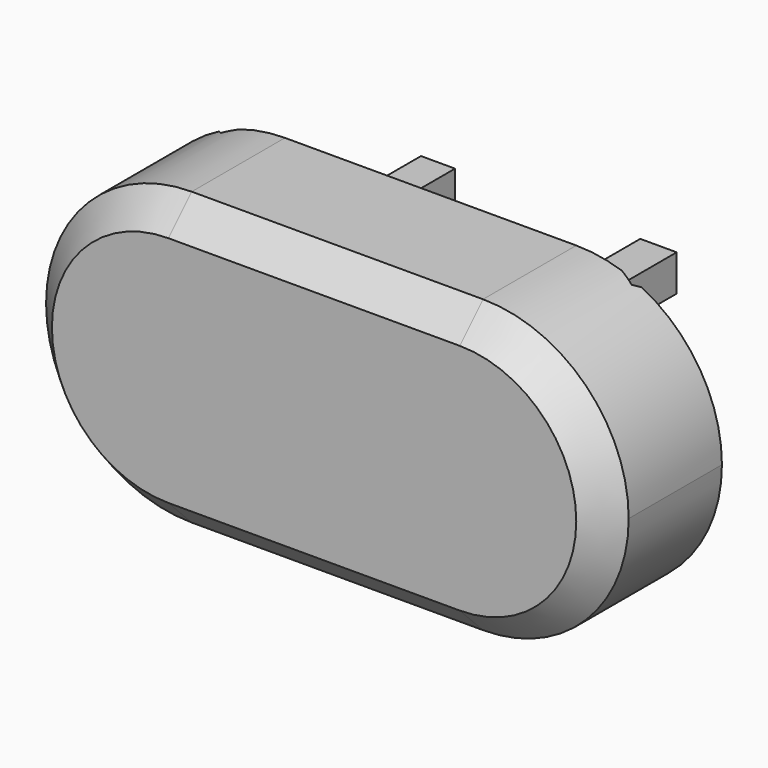
from build123d import *

# Parameters (mm, degrees)
F1_DEPTH     = 25.4
F2_W         = 63.5
F2_H         = 38.1
F3_DEPTH     = 12.7
F4_T1_DEPTH  = 63.5
F4_T3_DEPTH  = 38.1
F4_T5_DEPTH  = 50.8
F4_T8_ANGLE  = 180
F4_T10_ANGLE = 180
F4_T15_DEPTH = 76.5641495789
F4_S16_R     = 25.4
F4_T17_DEPTH = 40
F4_T21_DEPTH = 51.1641495789
F4_S22_R     = 25.4
F4_T23_DEPTH = 27
F4_T30_DEPTH = 76.5641495789
F4_S31_R     = 25.4
F4_T32_DEPTH = 40
F4_T36_DEPTH = 51.1641495789
F4_S37_R     = 25.4
F4_T38_DEPTH = 27
F4_T45_DEPTH = 51.1641495789
F4_S46_R     = 25.4
F4_T47_DEPTH = 27
F4_T51_DEPTH = 76.5641495789
F4_S52_R     = 25.4
F4_T53_DEPTH = 40
F4_T60_DEPTH = 76.5641495789
F4_S61_R     = 25.4
F4_T62_DEPTH = 40
F4_T66_DEPTH = 51.1641495789
F4_S67_R     = 25.4
F4_T68_DEPTH = 27
F5_W         = 6.35
F5_H         = 6.35
F5_W_2       = 5.9358693383
F5_H_2       = 6.4880426841
F5_W_3       = 5.79782274
F5_H_3       = 5.521739329
F5_W_4       = 5.9358680336
F5_H_4       = 6.6260866729
F6_DEPTH     = 25.4


# Not quite as in the source:
# - a fillet or chamfer that OpenCascade refuses, or shapes differently, is made with other operations: its cross-section is extruded or revolved along the edge and cut away or added


with BuildPart() as f1:
    # F0 (on Front) → F1 (new body)
    with BuildSketch(Plane.XZ):
        with BuildLine():
            ThreePointArc((-50.8, 0), (-43.3605122421, -17.9605122421), (-25.4, -25.4))
            Line((-25.4, -25.4), (25.4, -25.4))
            ThreePointArc((25.4, -25.4), (43.3605122421, -17.9605122421), (50.8, 0))
            ThreePointArc((50.8, 0), (43.3605122421, 17.9605122421), (25.4, 25.4))
            Line((25.4, 25.4), (-25.4, 25.4))
            ThreePointArc((-25.4, 25.4), (-43.3605122421, 17.9605122421), (-50.8, 0))
        make_face()
    extrude(amount=F1_DEPTH)

    # F2 (on Front) → F3 (cut)
    with BuildSketch(Plane.XZ):
        Rectangle(F2_W, F2_H)
    extrude(amount=F3_DEPTH, mode=Mode.SUBTRACT)

    # F4: chamfer of 5.08 on 8 edges, made by hand

    # F4_s2 → F4_t1 (cut)
    with BuildSketch(Plane.YZ.offset(-31.75)):
        Polygon((0, 24.13), (-5.08, 19.05), (0, 19.05), align=None)
        Polygon((0, -24.13), (-5.08, -19.05), (0, -19.05), align=None)
    extrude(amount=F4_T1_DEPTH, mode=Mode.SUBTRACT)

    # F4_s4 → F4_t3 (cut)
    with BuildSketch(Plane.XY.offset(-19.05)):
        Polygon((-36.83, 0), (-31.75, -5.08), (-31.75, 0), align=None)
        Polygon((36.83, 0), (31.75, -5.08), (31.75, 0), align=None)
    extrude(amount=F4_T3_DEPTH, mode=Mode.SUBTRACT)

    # F4_s6 → F4_t5 (cut)
    with BuildSketch(Plane.YZ.offset(-25.4)):
        Polygon((-20.32, 25.4), (-25.4, 20.32), (-25.4, 25.4), align=None)
        Polygon((-25.4, -20.32), (-20.32, -25.4), (-25.4, -25.4), align=None)
    extrude(amount=F4_T5_DEPTH, mode=Mode.SUBTRACT)

    # F4_s7 → F4_t8 (revolve, cut)
    with BuildSketch(Plane.YZ.offset(-25.4)):
        Polygon((-20.32, -25.4), (-25.4, -20.32), (-25.4, -25.4), align=None)
    revolve(axis=Axis((-25.4, -25.4, 0), (0, 1, 0)), revolution_arc=F4_T8_ANGLE, mode=Mode.SUBTRACT)

    # F4_s9 → F4_t10 (revolve, cut)
    with BuildSketch(Plane.YZ.offset(25.4)):
        Polygon((-25.4, 20.32), (-20.32, 25.4), (-25.4, 25.4), align=None)
    revolve(axis=Axis((25.4, -25.4, 0), (0, 1, 0)), revolution_arc=F4_T10_ANGLE, mode=Mode.SUBTRACT)


with BuildPart() as f4_tool13:
    # F4_s14 → F4_t15 (new body)
    with BuildSketch(Plane.YZ.offset(44.8141495789)):
        Polygon((0, 24.13), (-5.08, 19.05), (0, 19.05), align=None)
    extrude(amount=-F4_T15_DEPTH)

    # F4_s16 → F4_t17 (intersect, symmetric)
    with BuildSketch(Plane.XZ.offset(2.5)):
        with Locations((25.4, 0)):
            Circle(F4_S16_R)
    extrude(amount=F4_T17_DEPTH, both=True, mode=Mode.INTERSECT)

    split(bisect_by=Plane.YZ.offset(31.75), keep=Keep.TOP)


with BuildPart() as f4_tool19:
    # F4_s20 → F4_t21 (new body)
    with BuildSketch(Plane.XY.offset(-19.05)):
        Polygon((36.83, 0), (31.75, -5.08), (31.75, 0), align=None)
    extrude(amount=F4_T21_DEPTH)

    # F4_s22 → F4_t23 (intersect, symmetric)
    with BuildSketch(Plane.XZ.offset(2.5)):
        with Locations((25.4, 0)):
            Circle(F4_S22_R)
    extrude(amount=F4_T23_DEPTH, both=True, mode=Mode.INTERSECT)

    split(bisect_by=Plane.XY.offset(19.05), keep=Keep.TOP)


with BuildPart() as f4_tool13_1:
    add(f4_tool13.part)

    # F4_t25: intersect F4_tool19
    add(f4_tool19.part, mode=Mode.INTERSECT)


with BuildPart() as f1_1:
    add(f1.part)

    # F4_t11: cut F4_tool13
    add(f4_tool13_1.part, mode=Mode.SUBTRACT)


with BuildPart() as f4_tool28:
    # F4_s29 → F4_t30 (new body)
    with BuildSketch(Plane.YZ.offset(31.75)):
        Polygon((0, 24.13), (-5.08, 19.05), (0, 19.05), align=None)
    extrude(amount=-F4_T30_DEPTH)

    # F4_s31 → F4_t32 (intersect, symmetric)
    with BuildSketch(Plane.XZ.offset(2.5)):
        with Locations((-25.4, 0)):
            Circle(F4_S31_R)
    extrude(amount=F4_T32_DEPTH, both=True, mode=Mode.INTERSECT)

    split(bisect_by=Plane.YZ.offset(-31.75), keep=Keep.BOTTOM)


with BuildPart() as f4_tool34:
    # F4_s35 → F4_t36 (new body)
    with BuildSketch(Plane.XY.offset(32.1141495789)):
        Polygon((-36.83, 0), (-31.75, -5.08), (-31.75, 0), align=None)
    extrude(amount=-F4_T36_DEPTH)

    # F4_s37 → F4_t38 (intersect, symmetric)
    with BuildSketch(Plane.XZ.offset(2.5)):
        with Locations((-25.4, 0)):
            Circle(F4_S37_R)
    extrude(amount=F4_T38_DEPTH, both=True, mode=Mode.INTERSECT)

    split(bisect_by=Plane.XY.offset(19.05), keep=Keep.TOP)


with BuildPart() as f4_tool28_1:
    add(f4_tool28.part)

    # F4_t40: intersect F4_tool34
    add(f4_tool34.part, mode=Mode.INTERSECT)


with BuildPart() as f1_2:
    add(f1_1.part)

    # F4_t26: cut F4_tool28
    add(f4_tool28_1.part, mode=Mode.SUBTRACT)


with BuildPart() as f4_tool43:
    # F4_s44 → F4_t45 (new body)
    with BuildSketch(Plane.XY.offset(19.05)):
        Polygon((-36.83, 0), (-31.75, -5.08), (-31.75, 0), align=None)
    extrude(amount=-F4_T45_DEPTH)

    # F4_s46 → F4_t47 (intersect, symmetric)
    with BuildSketch(Plane.XZ.offset(2.5)):
        with Locations((-25.4, 0)):
            Circle(F4_S46_R)
    extrude(amount=F4_T47_DEPTH, both=True, mode=Mode.INTERSECT)

    split(bisect_by=Plane.XY.offset(-19.05), keep=Keep.BOTTOM)


with BuildPart() as f4_tool49:
    # F4_s50 → F4_t51 (new body)
    with BuildSketch(Plane.YZ.offset(-44.8141495789)):
        Polygon((0, -24.13), (-5.08, -19.05), (0, -19.05), align=None)
    extrude(amount=F4_T51_DEPTH)

    # F4_s52 → F4_t53 (intersect, symmetric)
    with BuildSketch(Plane.XZ.offset(2.5)):
        with Locations((-25.4, 0)):
            Circle(F4_S52_R)
    extrude(amount=F4_T53_DEPTH, both=True, mode=Mode.INTERSECT)

    split(bisect_by=Plane.YZ.offset(-31.75), keep=Keep.BOTTOM)


with BuildPart() as f4_tool43_1:
    add(f4_tool43.part)

    # F4_t55: intersect F4_tool49
    add(f4_tool49.part, mode=Mode.INTERSECT)


with BuildPart() as f1_3:
    add(f1_2.part)

    # F4_t41: cut F4_tool43
    add(f4_tool43_1.part, mode=Mode.SUBTRACT)


with BuildPart() as f4_tool58:
    # F4_s59 → F4_t60 (new body)
    with BuildSketch(Plane.YZ.offset(-31.75)):
        Polygon((0, -24.13), (-5.08, -19.05), (0, -19.05), align=None)
    extrude(amount=F4_T60_DEPTH)

    # F4_s61 → F4_t62 (intersect, symmetric)
    with BuildSketch(Plane.XZ.offset(2.5)):
        with Locations((25.4, 0)):
            Circle(F4_S61_R)
    extrude(amount=F4_T62_DEPTH, both=True, mode=Mode.INTERSECT)

    split(bisect_by=Plane.YZ.offset(31.75), keep=Keep.TOP)


with BuildPart() as f4_tool64:
    # F4_s65 → F4_t66 (new body)
    with BuildSketch(Plane.XY.offset(-32.1141495789)):
        Polygon((36.83, 0), (31.75, -5.08), (31.75, 0), align=None)
    extrude(amount=F4_T66_DEPTH)

    # F4_s67 → F4_t68 (intersect, symmetric)
    with BuildSketch(Plane.XZ.offset(2.5)):
        with Locations((25.4, 0)):
            Circle(F4_S67_R)
    extrude(amount=F4_T68_DEPTH, both=True, mode=Mode.INTERSECT)

    split(bisect_by=Plane.XY.offset(-19.05), keep=Keep.BOTTOM)


with BuildPart() as f4_tool58_1:
    add(f4_tool58.part)

    # F4_t70: intersect F4_tool64
    add(f4_tool64.part, mode=Mode.INTERSECT)


with BuildPart() as f1_4:
    add(f1_3.part)

    # F4_t56: cut F4_tool58
    add(f4_tool58_1.part, mode=Mode.SUBTRACT)

    # F5 (on Front) → F6 (join, symmetric)
    with BuildSketch(Plane.XZ):
        with Locations((19.4146236851, 9.9391293569)):
            Rectangle(F5_W, F5_H)
        with Locations((19.2075583543, -10.1461946878)):
            Rectangle(F5_W_2, F5_H_2)
        with Locations((-18.9614597259, -10.3532596925)):
            Rectangle(F5_W_3, F5_H_3)
        with Locations((-19.0304823727, 10.0771726934)):
            Rectangle(F5_W_4, F5_H_4)
    extrude(amount=F6_DEPTH, both=True)


solid = f1_4.part
